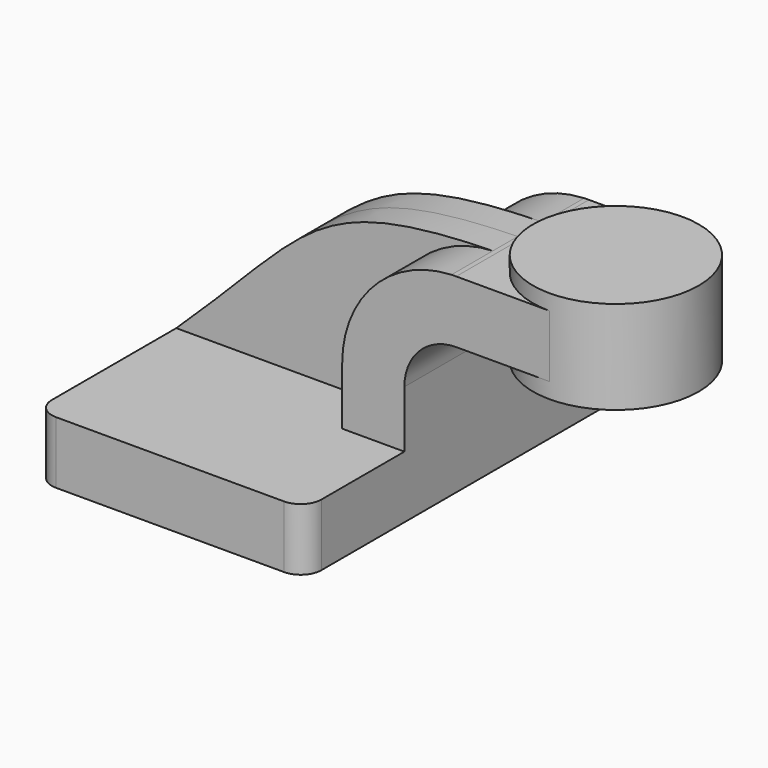
from build123d import *

# Parameters (mm, degrees)
F1_DEPTH = 63.5
F2_DEPTH = 25.4
F3_DEPTH = 9.525
F0_W     = 25.4
F0_H     = 19.05
F4_DEPTH = 25.4
F6_R     = 6.35


# Not quite as in the source:
# - a feature names something its author has since deleted; it is built from what else it names


with BuildPart() as f1:
    # F0 (on Front) → F1 (new body, symmetric)
    with BuildSketch(Plane.XZ):
        Polygon((22.225, 9.525), (-41.275, 9.525), (-41.275, -9.525), (41.275, -9.525), (41.275, 9.525), align=None)
    extrude(amount=F1_DEPTH, both=True)

    # F0 (on Front) → F2 (join, symmetric)
    with BuildSketch(Plane.XZ):
        with BuildLine():
            Line((22.225, 27.0002), (22.225, 9.525))
            Line((22.225, 9.525), (41.275, 9.525))
            Line((41.275, 9.525), (41.275, 27.0002))
            ThreePointArc((41.275, 27.0002), (45.9246798487, 38.2255201513), (57.15, 42.8752))
            Line((57.15, 42.8752), (60.325, 42.8752))
            Line((60.325, 42.8752), (60.325, 61.9252))
            Line((60.325, 61.9252), (57.15, 61.9252))
            add(Edge.make_bspline(
                [(55.6853928695, 61.894476765), (56.1693943217, 61.9055488515), (56.6575757113, 61.9157865575), (57.15, 61.9252)],
                knots=[110.5437742754, 110.5437742754, 110.5437742754, 110.5437742754, 111.5045361635, 111.5045361635, 111.5045361635, 111.5045361635], degree=3))
            ThreePointArc((55.6853928695, 61.894476765), (31.9417966821, 51.1725418494), (22.225, 27.0002))
        make_face()
    extrude(amount=F2_DEPTH, both=True)

    # F0 (on Front) → F3 (join, symmetric)
    with BuildSketch(Plane.XZ):
        with BuildLine():
            add(Edge.make_bspline(
                [(-41.275, 9.525), (-0.3556397641, 48.3007017864), (-0.003064316, 60.620539654), (55.6853928695, 61.894476765)],
                knots=[0, 0, 0, 0, 110.5437742754, 110.5437742754, 110.5437742754, 110.5437742754], degree=3))
            Line((-41.275, 9.525), (22.225, 9.525))
            Line((22.225, 9.525), (22.225, 27.0002))
            ThreePointArc((22.225, 27.0002), (31.9417966821, 51.1725418494), (55.6853928695, 61.894476765))
        make_face()
    extrude(amount=F3_DEPTH, both=True)

    # F0 (on Front) → F4 (join, symmetric)
    with BuildSketch(Plane.XZ):
        with Locations((73.025, 52.4002)):
            Rectangle(F0_W, F0_H)
    extrude(amount=F4_DEPTH, both=True)

    # F0 (on Front) → F5 (revolve)
    with BuildSketch(Plane.XZ):
        Polygon((85.725, 66.675), (85.725, 61.9252), (85.725, 42.8752), (85.725, 38.1), (111.125, 38.1), (111.125, 66.675), align=None)
    revolve(axis=Axis((85.725, 0, 52.3875), (0, 0, -1)))

    # F6
    f6_edges = [f1.edges().sort_by_distance(p)[0] for p in [
        (41.275, -63.5, 0),
        (-41.275, -63.5, 0),
        (41.275, 63.5, 0),
        (-41.275, 63.5, 0),
    ]]
    fillet(f6_edges, radius=F6_R)


solid = f1.part
